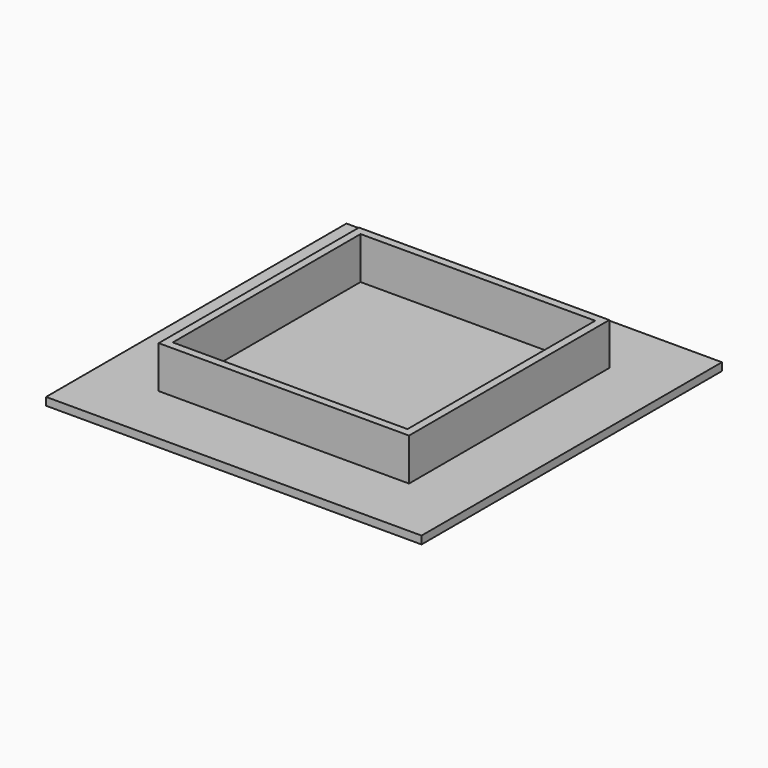
from build123d import *

# Parameters (mm, degrees)
F0_W     = 38.1
F0_H     = 38.1
F1_DEPTH = 0.79375
F2_W     = 25.4
F2_H     = 25.4
F4_DEPTH = 0.79375
F5_W     = 25.4
F5_H     = 25.4
F5_W_2   = 23.8125
F5_H_2   = 23.8125
F6_DEPTH = 5.08


with BuildPart() as f1:
    # F0 (on Top) → F1 (new body)
    with BuildSketch(Plane.XY):
        with Locations((-0.2852454782, 5.7126945901)):
            Rectangle(F0_W, F0_H)
    extrude(amount=F1_DEPTH)


with BuildPart() as f4:
    # F2 (on Top) → F4 (new body)
    with BuildSketch(Plane.XY):
        with Locations((-0.2852454782, 5.7126945901)):
            Rectangle(F2_W, F2_H)
    extrude(amount=-F4_DEPTH)

    # F5 (on face) → F6 (join)
    with BuildSketch(Plane.XY):
        with Locations((-0.2852454782, 5.7126945901)):
            Rectangle(F5_W, F5_H)
        with Locations((-0.2852454782, 5.7126945901)):
            Rectangle(F5_W_2, F5_H_2, mode=Mode.SUBTRACT)
    extrude(amount=F6_DEPTH)


solid = Compound([f1.part, f4.part])
